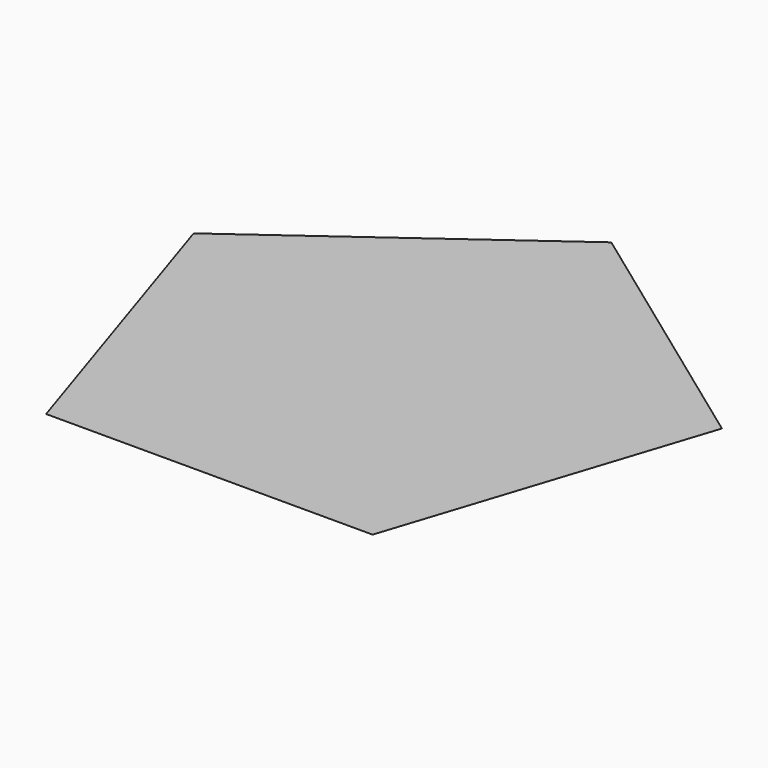
from build123d import *


# Not quite as in the source:
# - an extrude whose draft closes it to a point is written as a loft to that point


with BuildPart() as f1:
    # F0 (on Top) → F1 section 0
    with BuildSketch(Plane.XY, mode=Mode.PRIVATE) as f1_s0:
        Polygon((-221.450162536, -304.8), (221.450162536, -304.8), (358.3138897975, 116.423240229), (0, 376.7535195419), (-358.3138897975, 116.423240229), align=None)
    loft([f1_s0.sketch, Vertex(0, 0, -99.0355234118)], ruled=True)


solid = f1.part
